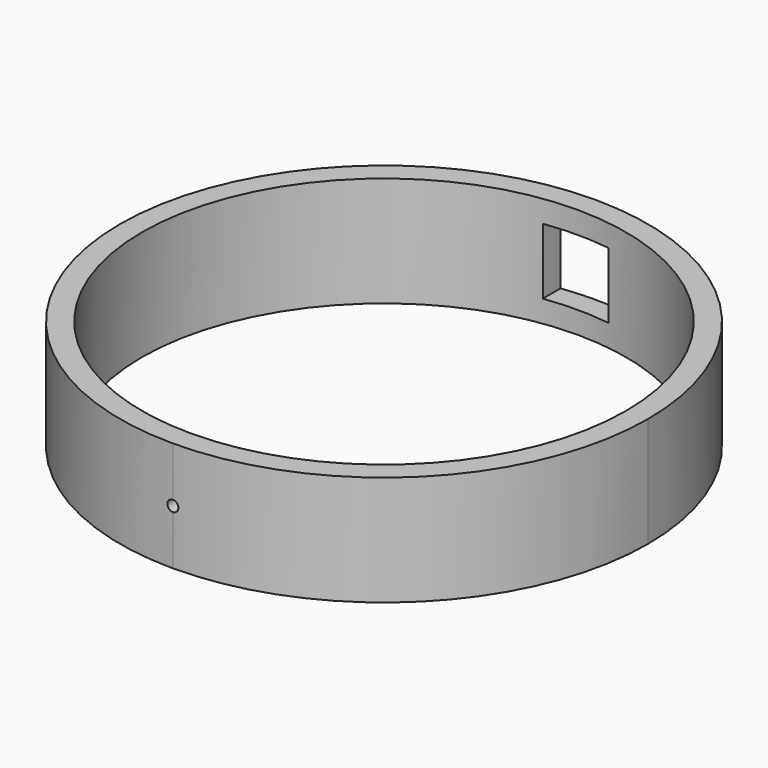
from build123d import *

# Parameters (mm, degrees)
F0_W        = 304.8
F0_H        = 304.8
F0_R        = 139.7
F1_DEPTH    = 63.5
F3_D        = 6.35
F2_W        = 38.1
F2_H        = 38.1
F2_R        = 1.5875
F4_DEPTH    = 25.4
F5_T1_DEPTH = 825.5


# Not quite as in the source:
# - a fillet or chamfer that OpenCascade refuses, or shapes differently, is made with other operations: its cross-section is extruded or revolved along the edge and cut away or added


with BuildPart() as f1:
    # F0 (on Top) → F1 (new body)
    with BuildSketch(Plane.XY):
        Rectangle(F0_W, F0_H)
        Circle(F0_R, mode=Mode.SUBTRACT)
    extrude(amount=F1_DEPTH)

    # F3 (through all)
    with Locations(Plane(origin=(0, 152.4, 0), x_dir=(-1, 0, 0), z_dir=(0, 1, 0))):
        with Locations((0, 31.75)):
            Hole(F3_D / 2)

    # F2 (on face) → F4 (cut)
    with BuildSketch(Plane(origin=(0, 152.4, 0), x_dir=(-1, 0, 0), z_dir=(0, 1, 0))):
        with Locations((0, 31.75)):
            Rectangle(F2_W, F2_H)
        with Locations((0, 31.75)):
            Circle(F2_R, mode=Mode.SUBTRACT)
    extrude(amount=-F4_DEPTH, mode=Mode.SUBTRACT)

    # F5: fillet of radius 152.4 on 4 edges, made by hand

    # F5_s2 → F5_t1 (cut)
    with BuildSketch(Plane.XY.offset(-381)):
        with BuildLine():
            ThreePointArc((0, 152.4), (-107.7630734528, 107.7630734528), (-152.4, 0))
            Line((-152.4, 0), (-152.4, 152.4))
            Line((-152.4, 152.4), (0, 152.4))
        make_face()
        with BuildLine():
            ThreePointArc((152.4, 0), (107.7630734528, 107.7630734528), (0, 152.4))
            Line((0, 152.4), (152.4, 152.4))
            Line((152.4, 152.4), (152.4, 0))
        make_face()
        with BuildLine():
            ThreePointArc((152.4, 0), (107.7630734528, -107.7630734528), (0, -152.4))
            Line((0, -152.4), (152.4, -152.4))
            Line((152.4, -152.4), (152.4, 0))
        make_face()
        with BuildLine():
            ThreePointArc((0, -152.4), (-107.7630734528, -107.7630734528), (-152.4, 0))
            Line((-152.4, 0), (-152.4, -152.4))
            Line((-152.4, -152.4), (0, -152.4))
        make_face()
    extrude(amount=F5_T1_DEPTH, mode=Mode.SUBTRACT)


solid = f1.part
